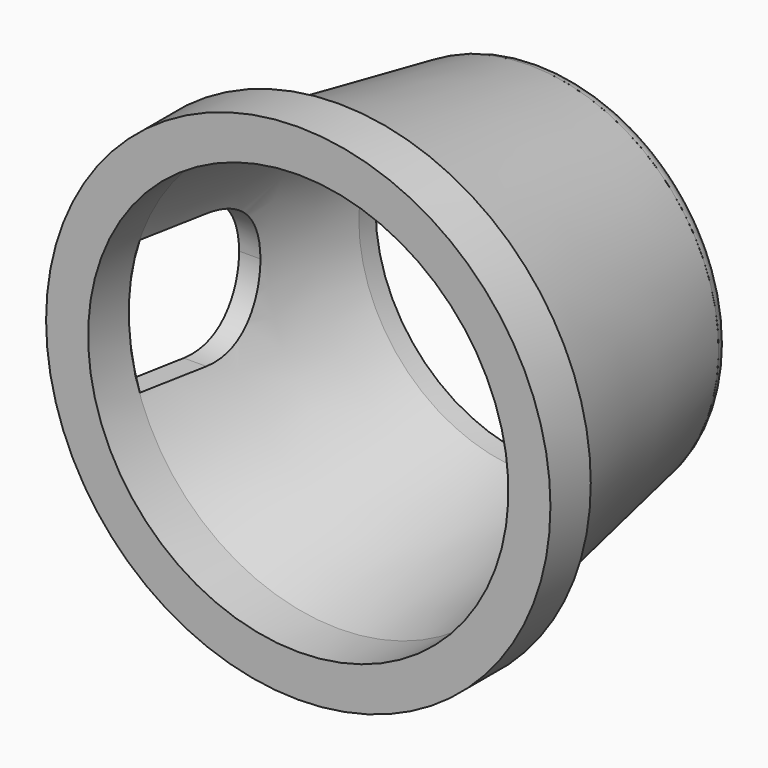
from build123d import *

# Parameters (mm, degrees)
F6_DEPTH = 38.1


with BuildPart() as f2:
    # F0 (on Right) → F2 (revolve)
    with BuildSketch(Plane.YZ):
        Polygon((-35.56, 31.75), (0, 25.4), (0.5401693397, 28.5287657554), (-35.56, 34.975224566), align=None)
    revolve(axis=Axis((0, -17.78, 0), (0, -1, 0)))

    # F1 (on Top) → F3 (revolve)
    with BuildSketch(Plane.XY):
        with BuildLine():
            Line((25.4, 3.175), (25.4, 0))
            Line((25.4, 0), (28.575, 0))
            ThreePointArc((28.575, 0), (27.6450640303, 2.2450640303), (25.4, 3.175))
        make_face()
    revolve(axis=Axis((0, 1.5875, 0), (0, 1, 0)))

    # F0 (on Right) → F4 (revolve)
    with BuildSketch(Plane.YZ):
        Polygon((-43.18, 31.75), (-35.56, 31.75), (-35.56, 34.975224566), (-35.56, 38.1), (-43.18, 38.1), align=None)
    revolve(axis=Axis((0, -39.37, 0), (0, -1, 0)))

    # F5 (on Right) → F6 (cut)
    with BuildSketch(Plane.YZ):
        with BuildLine():
            Line((-35.5086600387, 10.16), (-35.5086600387, 0))
            Line((-35.5086600387, 0), (-35.5086600387, -10.16))
            Line((-35.5086600387, -10.16), (-25.3486600387, -10.16))
            ThreePointArc((-25.3486600387, -10.16), (-18.1644551419, -7.1842048969), (-15.1886600387, 0))
            ThreePointArc((-15.1886600387, 0), (-18.1644551419, 7.1842048969), (-25.3486600387, 10.16))
            Line((-25.3486600387, 10.16), (-35.5086600387, 10.16))
        make_face()
    extrude(amount=-F6_DEPTH, mode=Mode.SUBTRACT)


solid = f2.part
